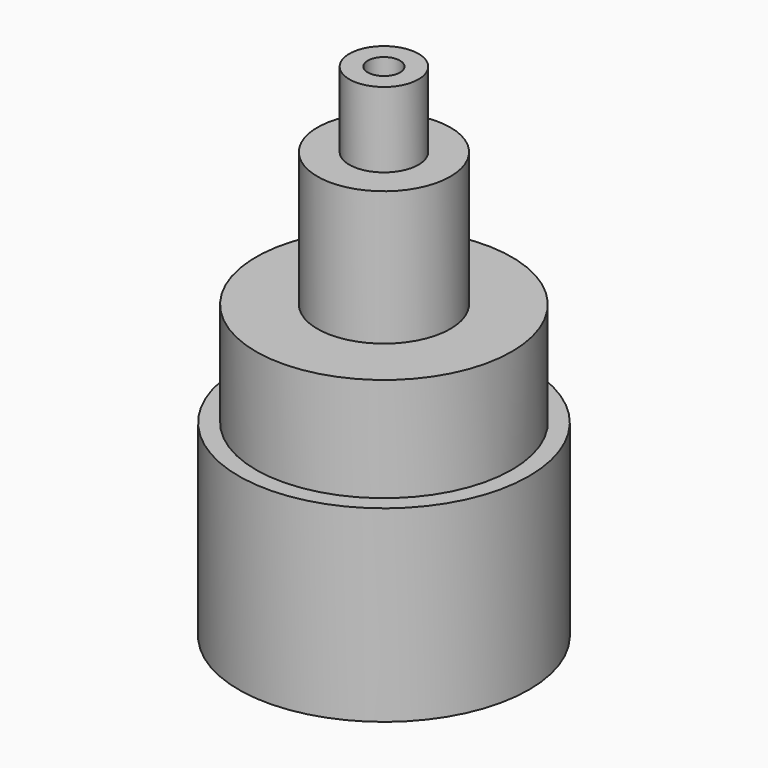
from build123d import *

# Parameters (mm, degrees)
F0_R     = 29.4132
F0_R_2   = 25.9334
F1_DEPTH = 38.1
F0_R_3   = 13.4736510141
F2_DEPTH = 59.182
F0_R_4   = 7.012968683
F3_DEPTH = 86.36
F4_DEPTH = 50.8
F0_R_5   = 3.2589999641
F5_DEPTH = 101.6


# Not quite as in the source:
# - the program builds the solid bodies; features that only make, move or delete a surface that nothing else refers to are left out


with BuildPart() as f1:
    # F0 (on Top) → F1 (new body)
    with BuildSketch(Plane.XY):
        Circle(F0_R)
        Circle(F0_R_2, mode=Mode.SUBTRACT)
    extrude(amount=F1_DEPTH)

    # F0 (on Top) → F2 (join)
    with BuildSketch(Plane.XY):
        Circle(F0_R_2)
        Circle(F0_R_3, mode=Mode.SUBTRACT)
    extrude(amount=F2_DEPTH)

    # F0 (on Top) → F3 (join)
    with BuildSketch(Plane.XY):
        Circle(F0_R_3)
        Circle(F0_R_4, mode=Mode.SUBTRACT)
    extrude(amount=F3_DEPTH)

    # F0 (on Top) → F4 (join)
    with BuildSketch(Plane.XY):
        Circle(F0_R_3)
        Circle(F0_R_4, mode=Mode.SUBTRACT)
    extrude(amount=F4_DEPTH)

    # F0 (on Top) → F5 (join)
    with BuildSketch(Plane.XY):
        Circle(F0_R_4)
        Circle(F0_R_5, mode=Mode.SUBTRACT)
    extrude(amount=F5_DEPTH)


solid = f1.part
